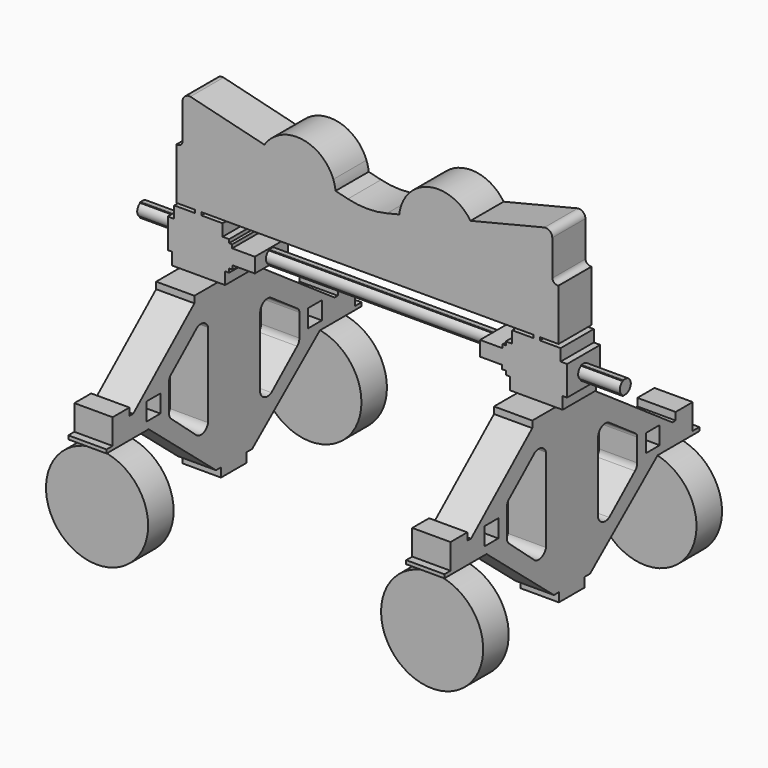
from build123d import *

# Parameters (mm, degrees)
F0_W      = 173.4239241437
F0_H      = 27.5425940983
F1_DEPTH  = 41.275
F0_W_2    = 77.2160674426
F3_DEPTH  = 6.35
F2_R      = 13.7068929279
F4_DEPTH  = 77.2160674426
F5_W      = 34.7150862217
F5_H      = 35.4616641998
F6_DEPTH  = 76.2
F10_DEPTH = 955.675
F11_R     = 12.7
F12_DEPTH = 127
F13_R     = 101.7419906729
F14_DEPTH = 63.5


with BuildPart() as f1:
    # F0 (on Front) → F1 (new body, symmetric)
    with BuildSketch(Plane.XZ):
        with BuildLine():
            Line((-330.5287990068, 0), (0, 0))
            Line((0, 0), (330.5287990068, 0))
            Line((330.5287990068, 0), (343.4204948115, 0))
            Line((343.4204948115, 0), (380.7005688964, 0))
            Line((380.7005688964, 0), (380.7005688964, 102.3223650141))
            ThreePointArc((380.7005688964, 102.3223650141), (372.5441671402, 104.1147287552), (368.2142413058, 111.2555410099))
            Line((368.2142413058, 111.2555410099), (368.2142413058, 182.2455618813))
            ThreePointArc((368.2142413058, 182.2455618813), (363.5014074864, 192.3735075188), (352.7182744195, 195.2907196651))
            Line((352.7182744195, 195.2907196651), (202.3475184069, 158.2654288336))
            ThreePointArc((202.3475184069, 158.2654288336), (211.8404844804, 138.1384042284), (215.097863992, 116.1247038796))
            ThreePointArc((215.097863992, 116.1247038796), (135.1035899776, 40.2148815001), (63.4864823908, 124.0741380534))
            Line((63.4864823908, 124.0741380534), (38.9052736437, 118.0215888278))
            ThreePointArc((38.9052736437, 118.0215888278), (0, 113.3023079411), (-38.9052736437, 118.0215888278))
            Line((-38.9052736437, 118.0215888278), (-63.581148316, 124.0974473291))
            ThreePointArc((-63.581148316, 124.0974473291), (-63.2728593455, 120.1163725983), (-63.170005363, 116.1247038796))
            ThreePointArc((-63.170005363, 116.1247038796), (-163.0602852006, 41.9188470477), (-205.2589334195, 158.9822968632))
            Line((-205.2589334195, 158.9822968632), (-352.7182744195, 195.2907196651))
            ThreePointArc((-352.7182744195, 195.2907196651), (-363.5014074864, 192.3735075188), (-368.2142413058, 182.2455618813))
            Line((-368.2142413058, 182.2455618813), (-368.2142413058, 111.2555410099))
            ThreePointArc((-368.2142413058, 111.2555410099), (-372.5441671402, 104.1147287552), (-380.7005688964, 102.3223650141))
            Line((-380.7005688964, 102.3223650141), (-380.7005688964, 0))
            Line((-380.7005688964, 0), (-343.4204948115, 0))
            Line((-343.4204948115, 0), (-330.5287990068, 0))
        make_face()
        with BuildLine():
            Line((-63.581148316, 124.0974473291), (-205.2589334195, 158.9822968632))
            ThreePointArc((-205.2589334195, 158.9822968632), (-163.0602852006, 41.9188470477), (-63.170005363, 116.1247038796))
            ThreePointArc((-63.170005363, 116.1247038796), (-63.2728593455, 120.1163725983), (-63.581148316, 124.0974473291))
        make_face()
        with BuildLine():
            ThreePointArc((215.097863992, 116.1247038796), (211.8404844804, 138.1384042284), (202.3475184069, 158.2654288336))
            Line((202.3475184069, 158.2654288336), (63.4864823908, 124.0741380534))
            ThreePointArc((63.4864823908, 124.0741380534), (135.1035899776, 40.2148815001), (215.097863992, 116.1247038796))
        make_face()
        with BuildLine():
            Line((63.4864823908, 124.0741380534), (202.3475184069, 158.2654288336))
            ThreePointArc((202.3475184069, 158.2654288336), (120.9098818399, 189.9342753539), (63.4864823908, 124.0741380534))
        make_face()
        with BuildLine():
            ThreePointArc((-63.581148316, 124.0974473291), (-122.1468943942, 191.3847827623), (-205.2589334195, 158.9822968632))
            Line((-205.2589334195, 158.9822968632), (-63.581148316, 124.0974473291))
        make_face()
        Polygon((343.4204948115, 0), (330.5287990068, 0), (330.5287990068, -5.919874861), (288.4773324014, -5.919874861), (288.4773324014, -29.554639552), (275.5856365967, -29.554639552), (275.5856365967, -36.6143758053), (269.446753087, -36.6143758053), (269.446753087, -43.6741086891), (224.3258312487, -43.6741086891), (224.3258312487, -45.4964258875), (397.7497553924, -45.4964258875), (397.7497553924, -29.554639552), (384.8580595877, -29.554639552), (384.8580595877, -5.919874861), (343.4204948115, -5.919874861), align=None)
        with Locations((311.0377933206, -59.2677229367)):
            Rectangle(F0_W, F0_H)
        Polygon((397.7497553924, -88.4880762434), (397.7497553924, -73.0390199858), (224.3258312487, -73.0390199858), (224.3258312487, -73.1408270348), (268.5259003434, -73.1408270348), (268.5259003434, -80.8144583781), (275.5856365967, -80.8144583781), (275.5856365967, -88.4880762434), (283.5661986374, -88.4880762434), (283.5661986374, -112.7367334972), (388.8483406081, -112.7367334972), (388.8483406081, -88.4880762434), align=None)
        with Locations((-311.0377933206, -59.2677229367)):
            Rectangle(F0_W, F0_H)
        Polygon((-330.5287990068, -5.919874861), (-330.5287990068, 0), (-343.4204948115, 0), (-343.4204948115, -5.919874861), (-384.8580595877, -5.919874861), (-384.8580595877, -29.554639552), (-397.7497553924, -29.554639552), (-397.7497553924, -45.4964258875), (-224.3258312487, -45.4964258875), (-224.3258312487, -43.6741086891), (-269.446753087, -43.6741086891), (-269.446753087, -36.6143758053), (-275.5856365967, -36.6143758053), (-275.5856365967, -29.554639552), (-288.4773324014, -29.554639552), (-288.4773324014, -5.919874861), align=None)
        Polygon((-224.3258312487, -73.0390199858), (-397.7497553924, -73.0390199858), (-397.7497553924, -88.4880762434), (-388.8483406081, -88.4880762434), (-388.8483406081, -112.7367334972), (-283.5661986374, -112.7367334972), (-283.5661986374, -88.4880762434), (-275.5856365967, -88.4880762434), (-275.5856365967, -80.8144583781), (-268.5259003434, -80.8144583781), (-268.5259003434, -73.1408270348), (-224.3258312487, -73.1408270348), align=None)
    extrude(amount=F1_DEPTH, both=True)

    # F0 (on Front) → F3 (join)
    with BuildSketch(Plane.XZ):
        with Locations((-436.3577891137, -59.2677229367)):
            Rectangle(F0_W_2, F0_H)
    extrude(amount=F3_DEPTH)

    # F2 (on face) → F4 (join, through all)
    with BuildSketch(Plane(origin=(-397.7497553924, 0, 0), x_dir=(0, -1, 0), z_dir=(-1, 0, 0))):
        with Locations((0, -59.0213578977)):
            Circle(F2_R)
    extrude(amount=F4_DEPTH)



with BuildPart() as f6:
    # F5 (on Right) → F6 (new body)
    with BuildSketch(Plane.YZ):
        Polygon((-32.8686577146, -571.1826070173), (0, -571.1826070173), (30.3709222289, -571.1826070173), (30.3709222289, -552.4953856619), (44.7580163796, -552.4953856619), (213.1403181177, -413.1031810811), (317.0471166506, -413.1031810811), (317.0471166506, -405.9177611568), (300.5285917146, -405.9177611568), (300.5285917146, -355.3389291226), (257.9001904089, -355.3389291226), (257.9001904089, -370.389823242), (249.9073350139, -370.389823242), (59.6779648766, -238.6435726777), (59.6779648766, -225.3222006197), (-99.1129318276, -225.3222006197), (-99.1129318276, -238.6435726777), (-251.6250382011, -370.389823242), (-260.80642746, -370.389823242), (-260.80642746, -355.6197680862), (-302.7214082854, -355.6197680862), (-302.7214082854, -405.9177611568), (-317.8906787482, -405.9177611568), (-317.8906787482, -413.1031810811), (-212.9035654309, -413.1031810811), (-45.2435617288, -553.2190438064), (-32.8686577146, -553.2190438064), align=None)
        with Locations((-200.9657472372, -379.881888628)):
            Rectangle(F5_W, F5_H, mode=Mode.SUBTRACT)
        with BuildLine():
            Line((-162.3312234879, -405.8248996735), (-162.3312234879, -378.5754144192))
            Line((-162.3312234879, -378.5754144192), (-162.3312234879, -351.3259291649))
            ThreePointArc((-162.3312234879, -351.3259291649), (-160.8619669011, -344.7298365867), (-156.7320078611, -339.3809497356))
            Line((-156.7320078611, -339.3809497356), (-92.6696360111, -284.0152084827))
            ThreePointArc((-92.6696360111, -284.0152084827), (-75.9611886995, -282.6286550171), (-64.7334083915, -295.0798273087))
            Line((-64.7334083915, -295.0798273087), (-64.7334083915, -378.5754144192))
            Line((-64.7334083915, -378.5754144192), (-64.7334083915, -462.0710015297))
            ThreePointArc((-64.7334083915, -462.0710015297), (-75.9611886995, -474.5221738212), (-92.6696360111, -473.1356203556))
            Line((-92.6696360111, -473.1356203556), (-156.7320078611, -417.7698791027))
            ThreePointArc((-156.7320078611, -417.7698791027), (-160.8619669011, -412.4209922516), (-162.3312234879, -405.8248996735))
        make_face(mode=Mode.SUBTRACT)
        with BuildLine():
            ThreePointArc((162.3312234879, -405.8248996735), (160.8619669011, -412.4209922516), (156.7320078611, -417.7698791027))
            Line((156.7320078611, -417.7698791027), (92.6696360111, -473.1356203556))
            ThreePointArc((92.6696360111, -473.1356203556), (75.9611886995, -474.5221738212), (64.7334083915, -462.0710015297))
            Line((64.7334083915, -462.0710015297), (64.7334083915, -321.9641149044))
            ThreePointArc((64.7334083915, -321.9641149044), (73.8183102497, -306.3218034571), (91.9069200754, -306.4616024494))
            Line((91.9069200754, -306.4616024494), (156.7356139421, -351.559817791))
            ThreePointArc((156.7356139421, -351.559817791), (160.8220673158, -355.3645627303), (162.3312234879, -360.7402145863))
            Line((162.3312234879, -360.7402145863), (162.3312234879, -405.8248996735))
        make_face(mode=Mode.SUBTRACT)
        with Locations((200.9657472372, -379.881888628)):
            Rectangle(F5_W, F5_H, mode=Mode.SUBTRACT)
    extrude(amount=F6_DEPTH)


with BuildPart() as f6_1:
    # F7: moved
    add(f6.part.moved(Location((298.45, 0, 0))))


with BuildPart() as f6_2:
    # F8: moved
    add(f6_1.part.moved(Location((0, 0, 112.5855))))


with BuildPart() as f1_1:
    add(f1.part)

    add(f6_2.part)  # F9 merges F6
    # F9: F6 across plane
    add(f6_2.part.mirror(Plane.YZ))

    # F10 (add): a face of the model
    f10_faces = [f1_1.faces().sort_by_distance(p)[0] for p in [
        (-474.965822835, -0.0562661704, -59.0872884251),
    ]]
    extrude(f10_faces, amount=-F10_DEPTH)

    # F11 (on face) → F12 (join)
    with BuildSketch(Plane(origin=(0, 0, -300.5176810811), x_dir=(1, 0, 0), z_dir=(0, 0, -1))):
        with Locations((336.55, 265.3971220895)):
            Circle(F11_R)
        with Locations((-336.55, -265.0937173842)):
            Circle(F11_R)
        with Locations((336.55, -265.0937173842)):
            Circle(F11_R)
        with Locations((-336.55, 265.3971220895)):
            Circle(F11_R)
    extrude(amount=F12_DEPTH)



with BuildPart() as f14:
    # F13 (on face) → F14 (new body)
    with BuildSketch(Plane(origin=(0, 300.5285917146, 0), x_dir=(-1, 0, 0), z_dir=(0, 1, 0))):
        with Locations((-390.9166753292, -413.5255813599)):
            Circle(F13_R)
    extrude(amount=F14_DEPTH)


with BuildPart() as f14_1:
    # F15: moved
    add(f14.part.moved(Location((0, -66.675, 0))))


with BuildPart() as f14_2:
    # F16: moved
    add(f14_1.part.moved(Location((-57.15, 0, 0))))


with BuildPart() as f1_2:
    add(f1_1.part)

    add(f14_2.part)  # F17 merges F14
    # F17: F14 across plane
    add(f14_2.part.mirror(Plane.XZ))

    # F18: F1 across plane


with BuildPart() as f1_3:
    add(f1_2.part)
    add(f1_2.part.mirror(Plane.YZ))


solid = f1_3.part
